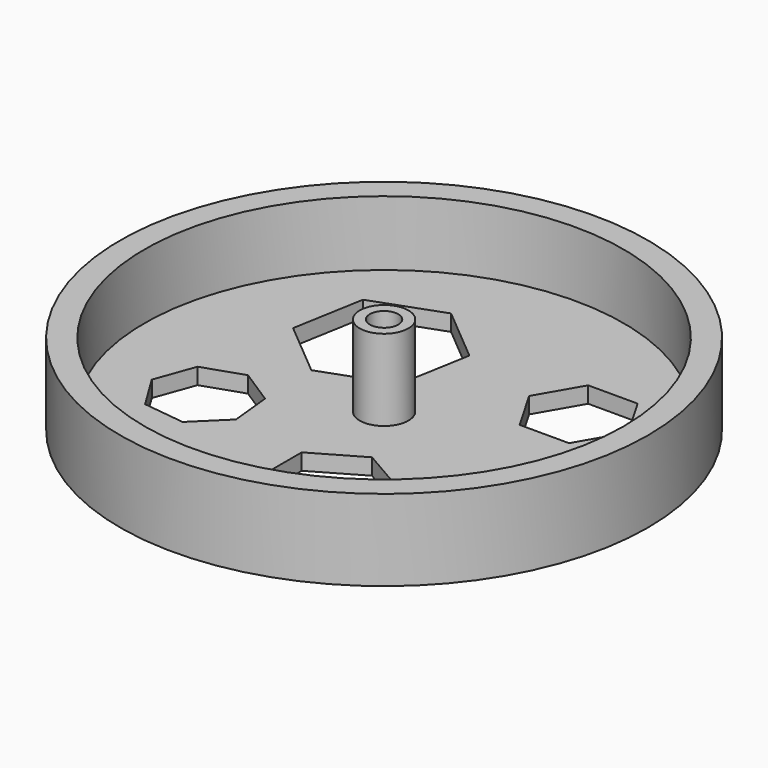
from build123d import *

# Parameters (mm, degrees)
F0_R      = 32.5
F1_DEPTH  = 10
F2_R      = 29.5
F3_DEPTH  = 8
F6_D      = 3.5
F8_DEPTH  = 2
F9_DEPTH  = 2
F10_DEPTH = 2
F11_DEPTH = 2
F4_R      = 3
F12_DEPTH = 10
F14_D     = 3.5


# Not quite as in the source:
# - the program builds the solid bodies; features that only make, move or delete a surface that nothing else refers to are left out


with BuildPart() as f1:
    # F0 (on Top) → F1 (new body)
    with BuildSketch(Plane.XY):
        Circle(F0_R)
    extrude(amount=F1_DEPTH)

    # F2 (on face) → F3 (cut)
    with BuildSketch(Plane.XY.offset(10)):
        Circle(F2_R)
    extrude(amount=-F3_DEPTH, mode=Mode.SUBTRACT)

    # F6 (through all)
    with Locations(Plane(origin=(0, 0, 0), x_dir=(1, 0, 0), z_dir=(0, 0, -1))):
        with Locations((0, 0)):
            Hole(F6_D / 2)

    # F7 (on face) → F8 (cut, through all)
    with BuildSketch(Plane.XY.offset(2)):
        Polygon((-7.741649435, 19.9890607288), (-16.1482516815, 16.9295235286), (-17.7019158656, 8.1194238235), (-10.8489778032, 2.3688613186), (-2.4423755567, 5.4283985188), (-0.8887113726, 14.2384982239), align=None)
    extrude(amount=-F8_DEPTH, mode=Mode.SUBTRACT)

    # F7 (on face) → F9 (cut, through all)
    with BuildSketch(Plane.XY.offset(2)):
        Polygon((-0.8887113726, -11.5674306203), (-0.8887113726, -18.4087138127), (5.0360136665, -21.8293554089), (10.9607387056, -18.4087138127), (10.9607387056, -11.5674306203), (5.0360136665, -8.1467890241), align=None)
    extrude(amount=-F9_DEPTH, mode=Mode.SUBTRACT)

    # F7 (on face) → F10 (cut, through all)
    with BuildSketch(Plane.XY.offset(2)):
        Polygon((-13.7885178521, -13.7792561938), (-10.1013832644, -10.1707357179), (-10.6237473641, -5.0381421005), (-14.9622593298, -2.2464230215), (-19.8499311619, -3.897799888), (-21.6062462804, -8.7487522375), (-18.9086635788, -13.1464140096), align=None)
    extrude(amount=-F10_DEPTH, mode=Mode.SUBTRACT)

    # F7 (on face) → F11 (cut, through all)
    with BuildSketch(Plane.XY.offset(2)):
        Polygon((11.8978734544, 5.9852199629), (17.9896090695, 5.9852199629), (21.0354768771, 11.2608177587), (17.9896090695, 16.5364155546), (11.8978734544, 16.5364155546), (8.8520056468, 11.2608177587), align=None)
    extrude(amount=-F11_DEPTH, mode=Mode.SUBTRACT)

    # F4 (on face) → F12 (join)
    with BuildSketch(Plane.XY.offset(2)):
        Circle(F4_R)
    extrude(amount=F12_DEPTH)

    # F14 (through all)
    with Locations(Plane.XY.offset(12)):
        with Locations((0, 0)):
            Hole(F14_D / 2)


solid = f1.part
